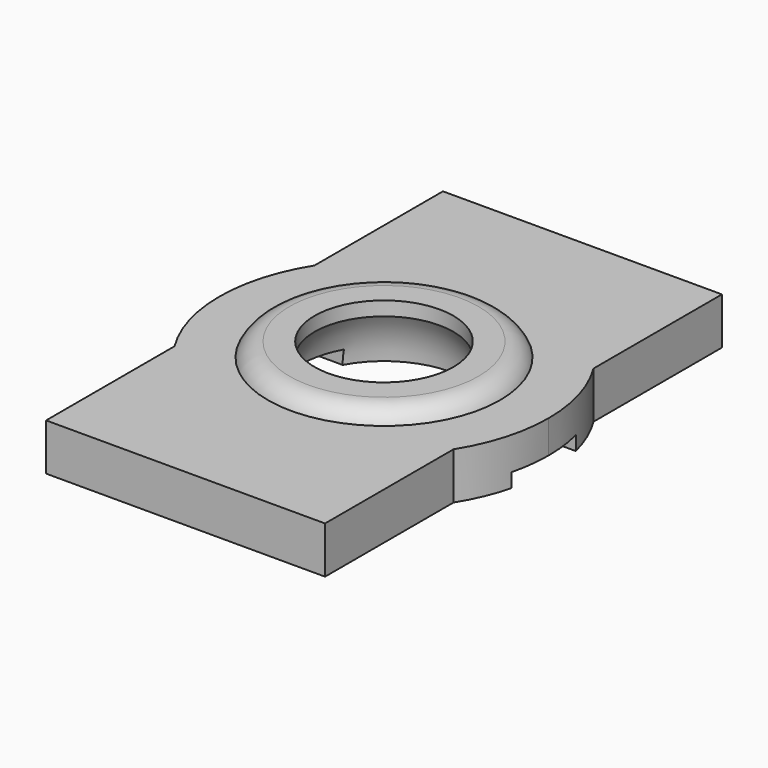
from build123d import *

# Parameters (mm, degrees)
F1_DEPTH = 10
F2_W     = 79.171128571
F2_H     = 17.1256698668
F3_DEPTH = 3
F6_R     = 24.75004298
F6_R_2   = 14.8028536267
F7_DEPTH = 3


# Not quite as in the source:
# - a fillet or chamfer that OpenCascade refuses, or shapes differently, is made with other operations: its cross-section is extruded or revolved along the edge and cut away or added


with BuildPart() as f1:
    # F0 (on Top) → F1 (new body)
    with BuildSketch(Plane.XY):
        with BuildLine():
            Line((-29.7593586147, -18.6613375429), (-29.7593586147, -52.9211238027))
            Line((-29.7593586147, -52.9211238027), (29.7593586147, -52.9211238027))
            Line((29.7593586147, -52.9211238027), (29.7593586147, -18.6613375429))
            ThreePointArc((29.7593586147, -18.6613375429), (0, -35.1264137658), (-29.7593586147, -18.6613375429))
        make_face()
        with BuildLine():
            ThreePointArc((-29.7593586147, 18.6613375429), (-35.1264137658, 0), (-29.7593586147, -18.6613375429))
            Line((-29.7593586147, -18.6613375429), (-29.7593586147, 18.6613375429))
        make_face()
        with BuildLine():
            Line((-29.7593586147, 18.6613375429), (-29.7593586147, -18.6613375429))
            ThreePointArc((-29.7593586147, -18.6613375429), (0, -35.1264137658), (29.7593586147, -18.6613375429))
            Line((29.7593586147, -18.6613375429), (29.7593586147, 18.6613375429))
            ThreePointArc((29.7593586147, 18.6613375429), (0, 35.1264137658), (-29.7593586147, 18.6613375429))
        make_face()
        with BuildLine():
            Line((29.7593586147, 18.6613375429), (29.7593586147, -18.6613375429))
            ThreePointArc((29.7593586147, -18.6613375429), (33.7579952615, -9.7088979792), (35.1264137658, 0))
            ThreePointArc((35.1264137658, 0), (33.7579952615, 9.7088979792), (29.7593586147, 18.6613375429))
        make_face()
        with BuildLine():
            Line((-29.7593586147, 52.9211238027), (-29.7593586147, 18.6613375429))
            ThreePointArc((-29.7593586147, 18.6613375429), (0, 35.1264137658), (29.7593586147, 18.6613375429))
            Line((29.7593586147, 18.6613375429), (29.7593586147, 52.9211238027))
            Line((29.7593586147, 52.9211238027), (-29.7593586147, 52.9211238027))
        make_face()
    extrude(amount=F1_DEPTH)

    # F2 (on Top) → F3 (cut)
    with BuildSketch(Plane.XY):
        Rectangle(F2_W, F2_H)
    extrude(amount=F3_DEPTH, mode=Mode.SUBTRACT)

    # F4 (on Front) → F5 (revolve, cut)
    with BuildSketch(Plane.XZ):
        with BuildLine():
            Line((0, -17.8640554044), (0, 17.8640554044))
            ThreePointArc((0, 17.8640554044), (-17.8640554044, 0), (0, -17.8640554044))
        make_face()
    revolve(axis=Axis((0, 0, 2.6136357337), (0, 0, 1)), mode=Mode.SUBTRACT)

    # F6 (on face) → F7 (join)
    with BuildSketch(Plane.XY.offset(10)):
        Circle(F6_R)
        Circle(F6_R_2, mode=Mode.SUBTRACT)
    extrude(amount=F7_DEPTH)

    # F8: fillet of radius 5 on 1 edges, made by hand

    # F8_s1 → F8_t2 (revolve, cut)
    with BuildSketch(Plane.XZ):
        with BuildLine():
            ThreePointArc((24.75004298, 10), (22.9060800725, 12.1833001327), (20.167467285, 13))
            Line((20.167467285, 13), (24.75004298, 13))
            Line((24.75004298, 13), (24.75004298, 10))
        make_face()
    revolve(axis=Axis((0, 0, 13), (0, 0, 1)), mode=Mode.SUBTRACT)


solid = f1.part
